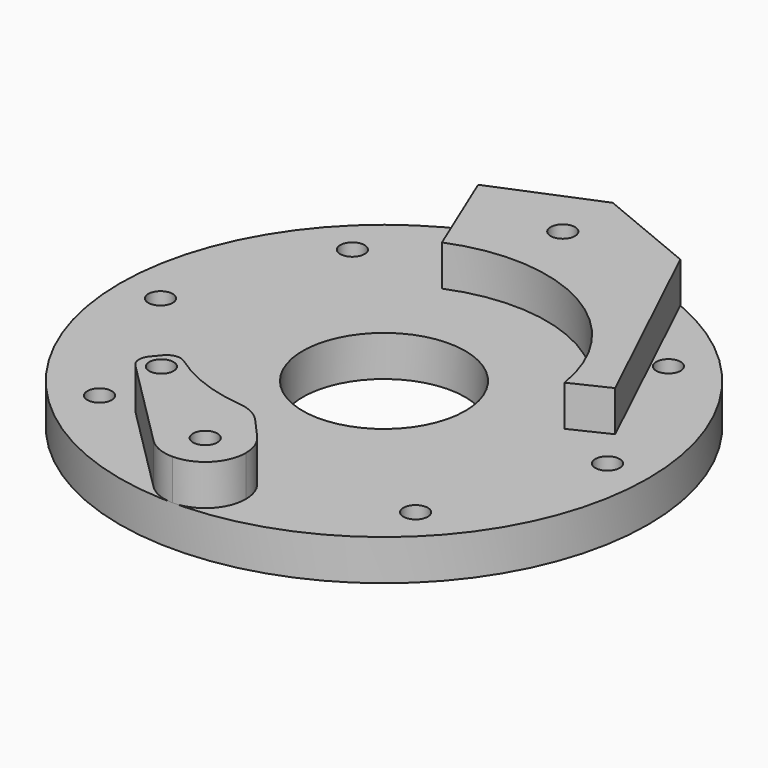
from build123d import *

# Parameters (mm, degrees)
F0_R     = 32.5
F0_R_2   = 1.5
F0_R_3   = 10
F1_DEPTH = 5
F2_R     = 1.5
F3_DEPTH = 5
F4_R     = 1.5
F5_DEPTH = 5
F6_R     = 1.7
F7_R     = 5


# Not quite as in the source:
# - a feature names something its author has since deleted; it is built from what else it names


with BuildPart() as f1:
    # F0 (on Top) → F1 (new body)
    with BuildSketch(Plane.XY):
        Circle(F0_R)
        with Locations((-19.4454364826, -19.4454364826)):
            Circle(F0_R_2, mode=Mode.SUBTRACT)
        with Locations((0, -27.5)):
            Circle(F0_R_2, mode=Mode.SUBTRACT)
        with Locations((19.4454364826, -19.4454364826)):
            Circle(F0_R_2, mode=Mode.SUBTRACT)
        with Locations((-27.5, 0)):
            Circle(F0_R_2, mode=Mode.SUBTRACT)
        with Locations((-19.4454364826, 19.4454364826)):
            Circle(F0_R_2, mode=Mode.SUBTRACT)
        Circle(F0_R_3, mode=Mode.SUBTRACT)
        with Locations((27.5, 0)):
            Circle(F0_R_2, mode=Mode.SUBTRACT)
        with Locations((0, 27.5)):
            Circle(F0_R_2, mode=Mode.SUBTRACT)
        with Locations((19.4454364826, 19.4454364826)):
            Circle(F0_R_2, mode=Mode.SUBTRACT)
    extrude(amount=F1_DEPTH)


with BuildPart() as f3:
    # F2 (on face) → F3 (new body)
    with BuildSketch(Plane.XY.offset(5)):
        with BuildLine():
            Line((12.4372115519, 30.0260848066), (0, 35.1777465095))
            Line((0, 35.1777465095), (-12.4372115519, 30.0260848066))
            ThreePointArc((-12.4372115519, 30.0260848066), (0, 32.5), (12.4372115519, 30.0260848066))
        make_face()
        with BuildLine():
            Line((24.2783450797, 5.2059809233), (12.4372115519, 30.0260848066))
            ThreePointArc((12.4372115519, 30.0260848066), (0, 32.5), (-12.4372115519, 30.0260848066))
            Line((-12.4372115519, 30.0260848066), (-7.6536686473, 18.4775906502))
            ThreePointArc((-7.6536686473, 18.4775906502), (9.8058067569, 17.4311833748), (19.7655989191, 3.0530475546))
            Line((19.7655989191, 3.0530475546), (24.2783450797, 5.2059809233))
        make_face()
        with Locations((0, 27.5)):
            Circle(F2_R, mode=Mode.SUBTRACT)
    extrude(amount=F3_DEPTH)


with BuildPart() as f3b:
    # F2 (on face) → F3, piece 2 (new body)
    with BuildSketch(Plane.XY.offset(5)):
        with BuildLine():
            ThreePointArc((0, -20), (-6.8404028665, -18.7938524157), (-12.8557521937, -15.3208888624))
            Line((-12.8557521937, -15.3208888624), (-16.0696902422, -19.151111078))
            ThreePointArc((-16.0696902422, -19.151111078), (-10.4611183934, -22.7060565039), (-4.1145152251, -24.6590909091))
            ThreePointArc((-4.1145152251, -24.6590909091), (-2.3233009432, -23.0725546048), (0, -22.5))
            Line((0, -22.5), (0, -20))
        make_face()
        with BuildLine():
            Line((3.7267799625, -24.1666666667), (0, -20))
            Line((0, -20), (0, -22.5))
            ThreePointArc((0, -22.5), (2.0412414523, -22.9356453541), (3.7267799625, -24.1666666667))
        make_face()
        with BuildLine():
            ThreePointArc((-4.1145152251, -24.6590909091), (-10.4611183934, -22.7060565039), (-16.0696902422, -19.151111078))
            Line((-16.0696902422, -19.151111078), (-16.0970617223, -19.1837311378))
            Line((-16.0970617223, -19.1837311378), (-3.4317429251, -31.1363636364))
            ThreePointArc((-3.4317429251, -31.1363636364), (-4.9724509563, -28.0241483443), (-4.1145152251, -24.6590909091))
        make_face()
        with BuildLine():
            ThreePointArc((3.7267799625, -24.1666666667), (2.0412414523, -22.9356453541), (0, -22.5))
            ThreePointArc((0, -22.5), (-2.3233009432, -23.0725546048), (-4.1145152251, -24.6590909091))
            ThreePointArc((-4.1145152251, -24.6590909091), (-4.9724509563, -28.0241483443), (-3.4317429251, -31.1363636364))
            ThreePointArc((-3.4317429251, -31.1363636364), (-1.8463723838, -32.1466018788), (-4.12e-08, -32.5))
            ThreePointArc((-4.12e-08, -32.5), (3.5355338914, -31.0355339205), (5, -27.5))
            ThreePointArc((5, -27.5), (4.6708617948, -25.7158895511), (3.7267799625, -24.1666666667))
        make_face()
        with Locations((0, -27.5)):
            Circle(F2_R, mode=Mode.SUBTRACT)
    extrude(amount=F3_DEPTH)

    # F4 (on face) → F5 (cut, through all)
    with BuildSketch(Plane.XY.offset(10)):
        Polygon((-3.4317429251, -31.1363636364), (-15.7756679175, -18.8007089162), (-16.0970617223, -19.1837311378), align=None)
        with Locations((-12.5758000287, -18.5207567512)):
            Circle(F4_R)
    extrude(amount=-F5_DEPTH, mode=Mode.SUBTRACT)

    # F6
    f6_edges = [f3b.edges().sort_by_distance(p)[0] for p in [
        (-15.775668, -18.800709, 7.5),
        (-12.855752, -15.320889, 7.5),
    ]]
    fillet(f6_edges, radius=F6_R)

    # F7
    f7_edges = [f3b.edges().sort_by_distance(p)[0] for p in [
        (0, -20, 7.5),
    ]]
    fillet(f7_edges, radius=F7_R)


solid = Compound([f1.part, f3.part, f3b.part])
